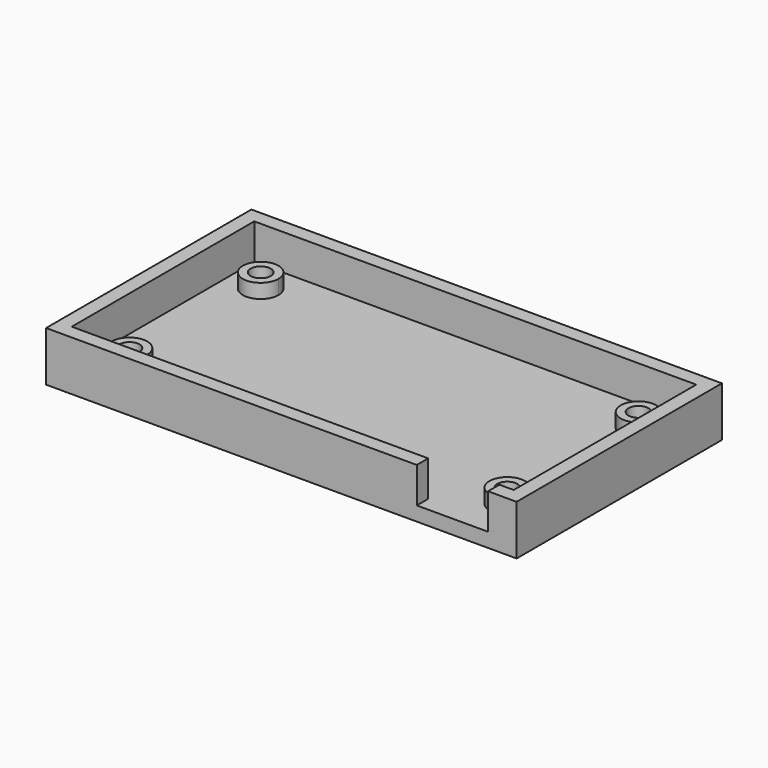
from build123d import *

# Parameters (mm, degrees)
F0_R     = 2.5
F0_R_2   = 1.4107797467
F0_W     = 10
F0_H     = 2
F1_DEPTH = 2
F2_DEPTH = 4
F3_DEPTH = 7


# Not quite as in the source:
# - a fillet or chamfer that OpenCascade refuses, or shapes differently, is made with other operations: its cross-section is extruded or revolved along the edge and cut away or added


with BuildPart() as f1:
    # F0 (on Top) → F1 (new body)
    with BuildSketch(Plane.XY):
        Polygon((19, -18), (19, -16), (10.7328139991, -16), (-31, -16), (-31, 16), (31, 16), (31, -16), (29, -16), (29, -18), (33, -18), (33, 18), (-33, 18), (-33, -18), align=None)
        Polygon((-30, -15), (-30, 15), (-26.5, 15), (30, 15), (30, -15), (29, -15), (29, -16), (31, -16), (31, 16), (-31, 16), (-31, -16), (10.7328139991, -16), (19, -16), (19, -15), align=None)
        Polygon((-26.5, 15), (-30, 15), (-30, -15), (19, -15), (24, -15), (29, -15), (30, -15), (30, 15), align=None)
        with Locations((-26.5, -11.5)):
            Circle(F0_R, mode=Mode.SUBTRACT)
        with Locations((26.5, -11.5)):
            Circle(F0_R, mode=Mode.SUBTRACT)
        with BuildLine():
            ThreePointArc((-24, 11.5), (-28.267766953, 9.732233047), (-26.5, 14))
            ThreePointArc((-26.5, 14), (-24.732233047, 13.267766953), (-24, 11.5))
        make_face(mode=Mode.SUBTRACT)
        with Locations((26.5, 11.5)):
            Circle(F0_R, mode=Mode.SUBTRACT)
        with BuildLine():
            ThreePointArc((-24, 11.5), (-24.732233047, 13.267766953), (-26.5, 14))
            ThreePointArc((-26.5, 14), (-28.267766953, 9.732233047), (-24, 11.5))
        make_face()
        with BuildLine():
            ThreePointArc((-25.0892202533, 11.5), (-27.4975719256, 10.5024280744), (-26.5, 12.9107797467))
            ThreePointArc((-26.5, 12.9107797467), (-25.5024280744, 12.4975719256), (-25.0892202533, 11.5))
        make_face(mode=Mode.SUBTRACT)
        with Locations((-26.5, -11.5)):
            Circle(F0_R)
        with Locations((-26.5, -11.5)):
            Circle(F0_R_2, mode=Mode.SUBTRACT)
        with Locations((26.5, -11.5)):
            Circle(F0_R)
        with Locations((26.5, -11.5)):
            Circle(F0_R_2, mode=Mode.SUBTRACT)
        with Locations((26.5, 11.5)):
            Circle(F0_R)
        with Locations((26.5, 11.5)):
            Circle(F0_R_2, mode=Mode.SUBTRACT)
        Polygon((24, -15), (19, -15), (19, -16), (29, -16), (29, -15), align=None)
        with Locations((24, -17)):
            Rectangle(F0_W, F0_H)
    extrude(amount=F1_DEPTH)

    # F0 (on Top) → F2 (join)
    with BuildSketch(Plane.XY):
        with Locations((-26.5, -11.5)):
            Circle(F0_R)
        with Locations((-26.5, -11.5)):
            Circle(F0_R_2, mode=Mode.SUBTRACT)
        with BuildLine():
            ThreePointArc((-24, 11.5), (-24.732233047, 13.267766953), (-26.5, 14))
            ThreePointArc((-26.5, 14), (-28.267766953, 9.732233047), (-24, 11.5))
        make_face()
        with BuildLine():
            ThreePointArc((-25.0892202533, 11.5), (-27.4975719256, 10.5024280744), (-26.5, 12.9107797467))
            ThreePointArc((-26.5, 12.9107797467), (-25.5024280744, 12.4975719256), (-25.0892202533, 11.5))
        make_face(mode=Mode.SUBTRACT)
        with Locations((26.5, -11.5)):
            Circle(F0_R)
        with Locations((26.5, -11.5)):
            Circle(F0_R_2, mode=Mode.SUBTRACT)
        with Locations((26.5, 11.5)):
            Circle(F0_R)
        with Locations((26.5, 11.5)):
            Circle(F0_R_2, mode=Mode.SUBTRACT)
    extrude(amount=F2_DEPTH)

    # F0 (on Top) → F3 (join)
    with BuildSketch(Plane.XY):
        Polygon((19, -18), (19, -16), (10.7328139991, -16), (-31, -16), (-31, 16), (31, 16), (31, -16), (29, -16), (29, -18), (33, -18), (33, 18), (-33, 18), (-33, -18), align=None)
    extrude(amount=F3_DEPTH)

    # F4: chamfer of 1.5 on 4 edges, made by hand

    # F4_s1 → F4_t2 (revolve, cut)
    with BuildSketch(Plane.XZ.offset(11.5)):
        with BuildLine():
            Line((29.4532061535, -0.0424264069), (27.8683533398, 1.5424264069))
            Line((27.8683533398, 1.5424264069), (27.8383533398, 1.5424264069))
            ThreePointArc((27.8383533398, 1.5424264069), (27.8807797467, 0.7712132034), (27.8807797467, 0))
            Line((27.8807797467, 0), (27.9107797467, -0.03))
            ThreePointArc((27.9107797467, -0.03), (28.6819929501, -0.03), (29.4532061535, -0.0724264069))
            Line((29.4532061535, -0.0724264069), (29.4532061535, -0.0424264069))
        make_face()
    revolve(axis=Axis((26.5, -11.5, 0), (0, 0, 1)), mode=Mode.SUBTRACT)

    # F4_s3 → F4_t4 (revolve, cut)
    with BuildSketch(Plane.XZ.offset(-11.5)):
        with BuildLine():
            Line((29.4532061535, -0.0424264069), (27.8683533398, 1.5424264069))
            Line((27.8683533398, 1.5424264069), (27.8383533398, 1.5424264069))
            ThreePointArc((27.8383533398, 1.5424264069), (27.8807797467, 0.7712132034), (27.8807797467, 0))
            Line((27.8807797467, 0), (27.9107797467, -0.03))
            ThreePointArc((27.9107797467, -0.03), (28.6819929501, -0.03), (29.4532061535, -0.0724264069))
            Line((29.4532061535, -0.0724264069), (29.4532061535, -0.0424264069))
        make_face()
    revolve(axis=Axis((26.5, 11.5, 0), (0, 0, 1)), mode=Mode.SUBTRACT)

    # F4_s5 → F4_t6 (revolve, cut)
    with BuildSketch(Plane.XZ.offset(-11.5)):
        with BuildLine():
            Line((-23.5467938465, -0.0424264069), (-25.1316466602, 1.5424264069))
            Line((-25.1316466602, 1.5424264069), (-25.1616466602, 1.5424264069))
            ThreePointArc((-25.1616466602, 1.5424264069), (-25.1192202533, 0.7712132034), (-25.1192202533, 0))
            Line((-25.1192202533, 0), (-25.0892202533, -0.03))
            ThreePointArc((-25.0892202533, -0.03), (-24.3180070499, -0.03), (-23.5467938465, -0.0724264069))
            Line((-23.5467938465, -0.0724264069), (-23.5467938465, -0.0424264069))
        make_face()
    revolve(axis=Axis((-26.5, 11.5, 0), (0, 0, 1)), mode=Mode.SUBTRACT)

    # F4_s7 → F4_t8 (revolve, cut)
    with BuildSketch(Plane.XZ.offset(11.5)):
        with BuildLine():
            Line((-23.5467938465, -0.0424264069), (-25.1316466602, 1.5424264069))
            Line((-25.1316466602, 1.5424264069), (-25.1616466602, 1.5424264069))
            ThreePointArc((-25.1616466602, 1.5424264069), (-25.1192202533, 0.7712132034), (-25.1192202533, 0))
            Line((-25.1192202533, 0), (-25.0892202533, -0.03))
            ThreePointArc((-25.0892202533, -0.03), (-24.3180070499, -0.03), (-23.5467938465, -0.0724264069))
            Line((-23.5467938465, -0.0724264069), (-23.5467938465, -0.0424264069))
        make_face()
    revolve(axis=Axis((-26.5, -11.5, 0), (0, 0, 1)), mode=Mode.SUBTRACT)


solid = f1.part
